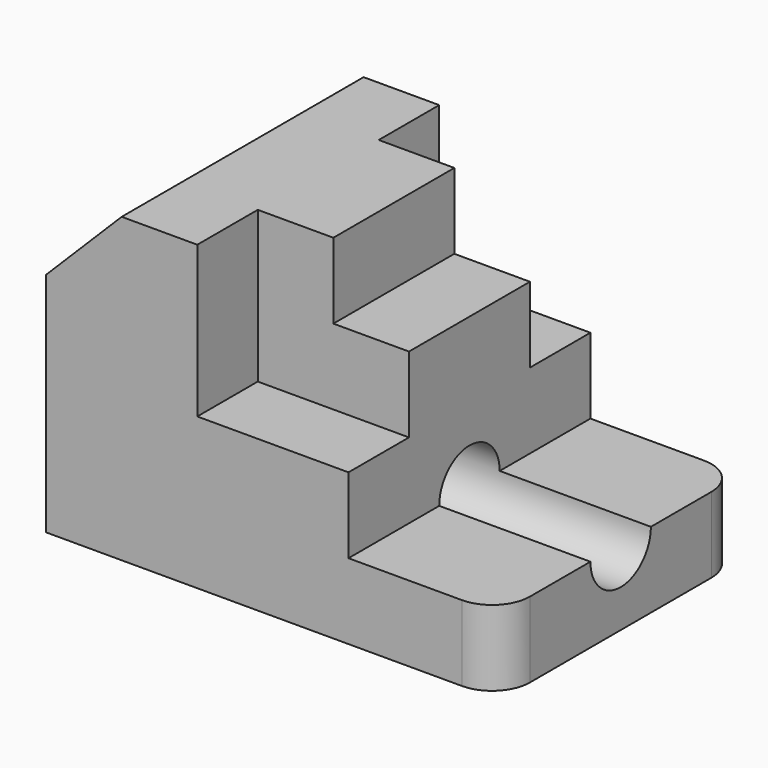
from build123d import *

# Parameters (mm, degrees)
F1_DEPTH  = 25.4
F2_DEPTH  = 50.8
F0_W      = 12.7
F0_H      = 50.8
F3_DEPTH  = 50.8
F4_DEPTH  = 25.4
F5_DEPTH  = 12.7
F7_DEPTH  = 50.801
F8_DEPTH  = 38.1
F0_W_2    = 25.4
F0_H_2    = 12.7
F9_DEPTH  = 12.7
F10_DEPTH = 148
F11_DEPTH = 50.801
F12_DEPTH = 12.7
F13_R     = 6.35
F14_DEPTH = 76.201


# Not quite as in the source:
# - an extrude ends at something that could not be found from the text; its depth is read off the source's solid


with BuildPart() as f1:
    # F0 (on Top) → F1 (new body)
    with BuildSketch(Plane.XY):
        Polygon((25.4, 12.7), (25.4, 0), (50.8, 0), (50.8, 12.7), (38.1, 12.7), align=None)
    extrude(amount=F1_DEPTH)

    # F0 (on Top) → F2 (join)
    with BuildSketch(Plane.XY):
        Polygon((12.7, 50.8), (12.7, 0), (25.4, 0), (25.4, 12.7), (38.1, 12.7), (38.1, 38.1), (25.4, 38.1), (25.4, 50.8), align=None)
    extrude(amount=F2_DEPTH)

    # F0 (on Top) → F3 (join)
    with BuildSketch(Plane.XY):
        with Locations((6.35, 25.4)):
            Rectangle(F0_W, F0_H)
    extrude(amount=F3_DEPTH)

    # F0 (on Top) → F4 (join)
    with BuildSketch(Plane.XY):
        Polygon((50.8, 50.8), (25.4, 50.8), (25.4, 38.1), (38.1, 38.1), (50.8, 38.1), align=None)
    extrude(amount=F4_DEPTH)

    # F0 (on Top) → F5 (join)
    with BuildSketch(Plane.XY):
        with BuildLine():
            Line((50.8, 12.7), (50.8, 0))
            Line((50.8, 0), (69.85, 0))
            ThreePointArc((69.85, 0), (74.3401280605, 1.8598719395), (76.2, 6.35))
            Line((76.2, 6.35), (76.2, 19.05))
            Line((76.2, 19.05), (50.8, 19.05))
            Line((50.8, 19.05), (50.8, 12.7))
        make_face()
        with BuildLine():
            Line((69.85, 50.8), (50.8, 50.8))
            Line((50.8, 50.8), (50.8, 38.1))
            Line((50.8, 38.1), (50.8, 31.75))
            Line((50.8, 31.75), (76.2, 31.75))
            Line((76.2, 31.75), (76.2, 44.45))
            ThreePointArc((76.2, 44.45), (74.3401280605, 48.9401280605), (69.85, 50.8))
        make_face()
    extrude(amount=F5_DEPTH)

    # F6 (on face) → F7 (cut, through all)
    with BuildSketch(Plane.XZ):
        Polygon((12.7, 50.8), (0, 50.8), (0, 38.1), align=None)
    extrude(amount=-F7_DEPTH, mode=Mode.SUBTRACT)

    # F0 (on Top) → F8 (join)
    with BuildSketch(Plane.XY):
        Polygon((38.1, 12.7), (50.8, 12.7), (50.8, 19.05), (50.8, 31.75), (50.8, 38.1), (38.1, 38.1), align=None)
    extrude(amount=F8_DEPTH)

    # F0 (on Top) → F9 (join)
    with BuildSketch(Plane.XY):
        with Locations((63.5, 25.4)):
            Rectangle(F0_W_2, F0_H_2)
    extrude(amount=F9_DEPTH)

    # F0 (on Top) → F10 (cut, through all)
    with BuildSketch(Plane.XY):
        with Locations((63.5, 25.4)):
            Rectangle(F0_W_2, F0_H_2)
    extrude(amount=-F10_DEPTH, mode=Mode.SUBTRACT)

    # F0 (on Top) → F11 (cut, through all)
    with BuildSketch(Plane.XY):
        with Locations((63.5, 25.4)):
            Rectangle(F0_W_2, F0_H_2)
    extrude(amount=F11_DEPTH, mode=Mode.SUBTRACT)

    # F0 (on Top) → F12 (join)
    with BuildSketch(Plane.XY):
        with Locations((63.5, 25.4)):
            Rectangle(F0_W_2, F0_H_2)
    extrude(amount=F12_DEPTH)

    # F13 (on face) → F14 (cut, through all)
    with BuildSketch(Plane.YZ.offset(76.2)):
        with Locations((25.4, 12.7)):
            Circle(F13_R)
    extrude(amount=-F14_DEPTH, mode=Mode.SUBTRACT)


solid = f1.part
